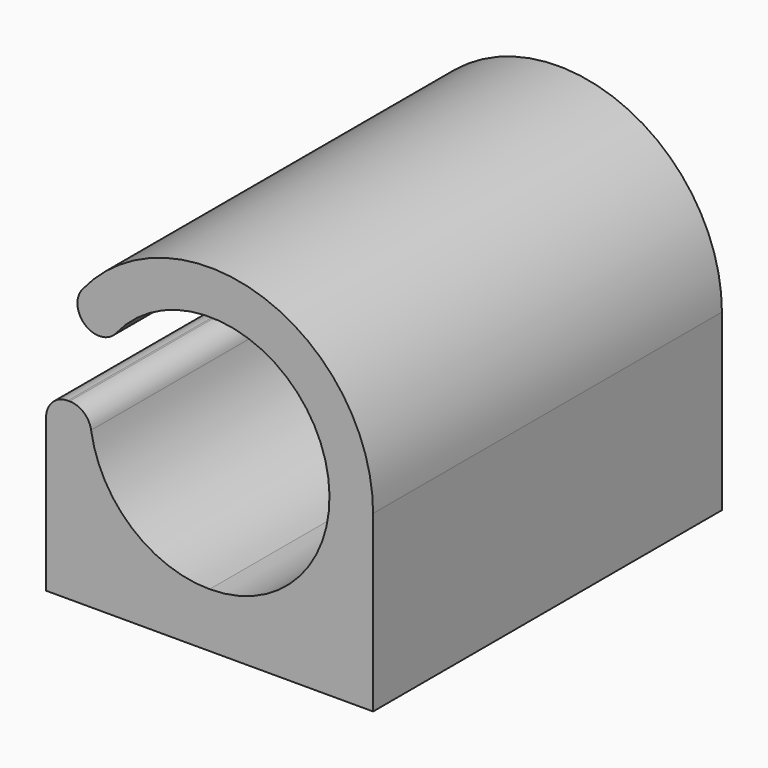
from build123d import *

# Parameters (mm, degrees)
F0_W         = 19.05
F0_H         = 25.4
F1_DEPTH     = 3.175
F3_DEPTH     = 25.4
F4_R         = 1.26999
F6_TEXT_SIZE = 8.3332051775
F7_DEPTH     = 1.27


# Not quite as in the source:
# - a fillet or chamfer is up to 0.001 mm smaller than in the source, because OpenCascade refuses the exact size
# - Text() gives the source's letters only with a copy of the font that has no kerning and outlines rounded to 1/6400 em; it was checked with that copy


with BuildPart() as f1:
    # F0 (on Top) → F1 (new body)
    with BuildSketch(Plane.XY):
        with Locations((9.525, 12.7)):
            Rectangle(F0_W, F0_H)
    extrude(amount=F1_DEPTH)

    # F2 (on face) → F3 (join, through all)
    with BuildSketch(Plane.XZ):
        with BuildLine():
            Line((9.525, 3.175), (19.05, 3.175))
            Line((19.05, 3.175), (19.05, 10.16))
            ThreePointArc((19.05, 10.16), (11.9902514046, 19.3604434954), (1.276108029, 14.9225))
            Line((1.276108029, 14.9225), (3.4758125546, 13.6525))
            ThreePointArc((3.4758125546, 13.6525), (15.5741874454, 13.6525), (9.525, 3.175))
        make_face()
        with BuildLine():
            Line((0, 3.175), (9.525, 3.175))
            ThreePointArc((9.525, 3.175), (4.5858591334, 5.2208591334), (2.54, 10.16))
            Line((2.54, 10.16), (0, 10.16))
            Line((0, 10.16), (0, 3.175))
        make_face()
    extrude(amount=-F3_DEPTH)

    # F4 (radius 1.27 in the source; OpenCascade refuses exactly that, so slightly less here)
    f4_edges = [f1.edges().sort_by_distance(p)[0] for p in [
        (1.276108, 12.7, 14.9225),
        (3.475813, 12.7, 13.6525),
        (2.54, 12.7, 10.16),
        (0, 12.7, 10.16),
    ]]
    fillet(f4_edges, radius=F4_R)

    # F6 (on face) → F7 (cut)
    with BuildSketch(Plane(origin=(0, 0, 0), x_dir=(0, -1, 0), z_dir=(-1, 0, 0))):
        with Locations((-17.78, 1.6200922722)):
            Text('TC', F6_TEXT_SIZE, font='Open Sans', text_align=(TextAlign.LEFT, TextAlign.BOTTOM))
    extrude(amount=-F7_DEPTH, mode=Mode.SUBTRACT)


solid = f1.part
